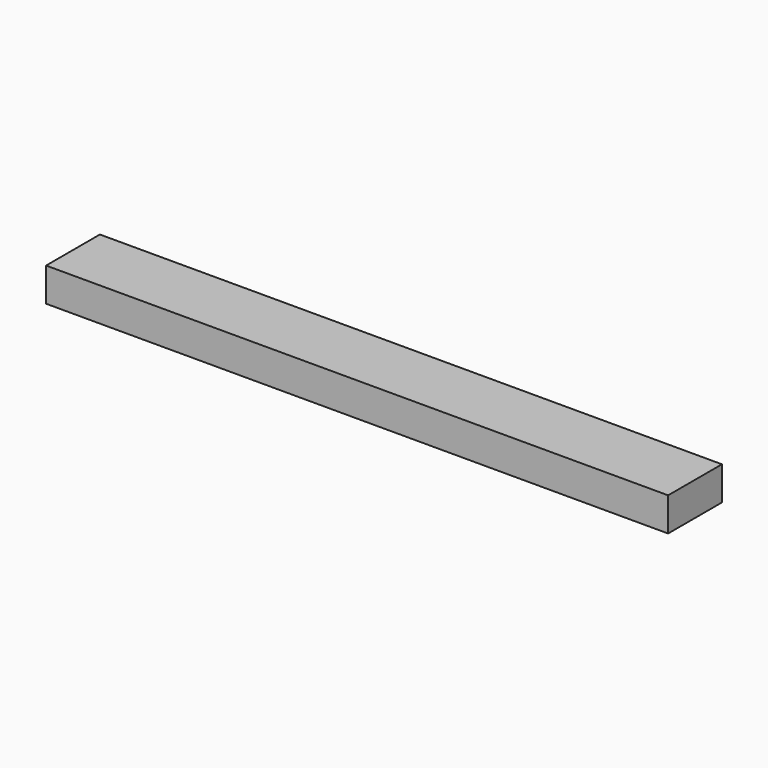
from build123d import *

# Parameters (mm, degrees)
F0_W     = 200
F0_H     = 100
F1_DEPTH = 1709


# Not quite as in the source:
# - a pattern or mirror of a feature is missing from the dataset's text; its kind, count and spacing are read off the source's solid


with BuildPart() as f1:
    # F0 (on Right) → F1 (new body)
    with BuildSketch(Plane.YZ):
        with Locations((-100, 50)):
            Rectangle(F0_W, F0_H)
    extrude(amount=F1_DEPTH)

    # F1_copies: F1 across plane


with BuildPart() as f1_1:
    add(f1.part)
    add(f1.part.mirror(Plane(origin=(925, 0, 0), x_dir=(0, 0, 1), z_dir=(1, 0, 0))))


solid = f1_1.part
